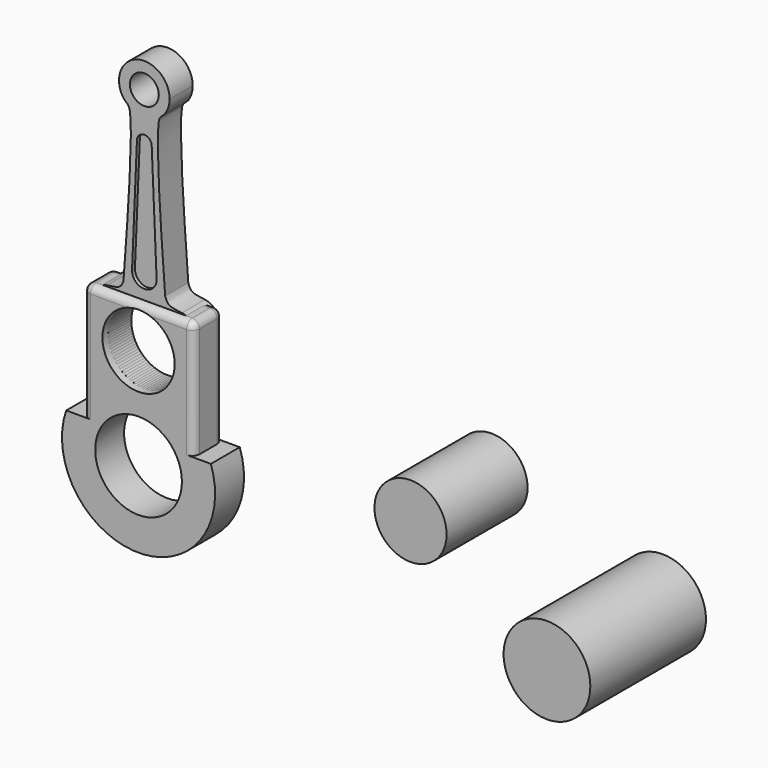
from build123d import *

# Parameters (mm, degrees)
F0_R          = 10
F1_DEPTH      = 20
F3_DEPTH      = 20
F5_DEPTH      = 2.5
F7_DEPTH      = 2.5
F8_R          = 30
F8_R_2        = 25
F9_DEPTH      = 25
F10_R         = 24.95
F11_DEPTH     = 35
F12_R         = 30
F13_DEPTH     = 100
F14_T1_DEPTH  = 66.4988437295
F14_T3_DEPTH  = 76.3163360927
F14_T6_ANGLE  = 90
F14_T8_ANGLE  = 90
F14_T10_ANGLE = 90
F14_T12_ANGLE = 90
F15_T1_DEPTH  = 69.8025602819


# Not quite as in the source:
# - a fillet or chamfer that OpenCascade refuses, or shapes differently, is made with other operations: its cross-section is extruded or revolved along the edge and cut away or added


with BuildPart() as f1:
    # F0 (on Front) → F1 (new body)
    with BuildSketch(Plane.XZ):
        with BuildLine():
            ThreePointArc((10.657655781, -13.8803592624), (0, -17.5), (-10.657655781, -13.8803592624))
            add(Edge.make_bspline(
                [(-10.657655781, -13.8803592624), (-10.5697063214, -14.0734920796), (-7.4212070748, -22.3661273448), (-11.0149524319, -76.0143110226), (-14.4087837187, -120.986558497)],
                knots=[0.171455294, 0.171455294, 0.171455294, 0.171455294, 0.1930861601, 1, 1, 1, 1], degree=3))
            add(Edge.make_bspline(
                [(-14.4087837187, -120.986558497), (-15, -122.5373980972), (-16.0166076681, -126.7545271526), (-23.3016373721, -127.0844308904), (-25.8878060456, -127.5592148304)],
                knots=[0, 0, 0, 0, 0.4297687598, 1, 1, 1, 1], degree=3))
            Line((-25.8878060456, -127.5592148304), (-35, -127.5592148304))
            Line((-35, -127.5592148304), (-35, -157.0267379284))
            Line((-35, -157.0267379284), (-25, -157.0267379284))
            ThreePointArc((-25, -157.0267379284), (0, -132.0267379284), (25, -157.0267379284))
            Line((25, -157.0267379284), (35, -157.0267379284))
            Line((35, -157.0267379284), (35, -127.5592148304))
            Line((35, -127.5592148304), (25.8878060456, -127.5592148304))
            add(Edge.make_bspline(
                [(14.4087837187, -120.986558497), (15, -122.5373980972), (16.0166076681, -126.7545271526), (23.3016373721, -127.0844308904), (25.8878060456, -127.5592148304)],
                knots=[0, 0, 0, 0, 0.4297687598, 1, 1, 1, 1], degree=3))
            add(Edge.make_bspline(
                [(10.657655781, -13.8803592624), (10.5697063214, -14.0734920796), (7.4212070748, -22.3661273448), (11.0149524319, -76.0143110226), (14.4087837187, -120.986558497)],
                knots=[0.171455294, 0.171455294, 0.171455294, 0.171455294, 0.1930861601, 1, 1, 1, 1], degree=3))
        make_face()
        with BuildLine():
            ThreePointArc((14.4087837187, -9.9316137535), (16.7093344433, -5.2007828701), (17.5, 0))
            ThreePointArc((17.5, 0), (-5.2007828701, 16.7093344433), (-14.4087837187, -9.9316137535))
            add(Edge.make_bspline(
                [(-14.4087837187, -9.9316137535), (-12.4132538877, -12.2865411794), (-11.3547799907, -12.3495077572), (-10.657655781, -13.8803592624)],
                knots=[0, 0, 0, 0, 0.171455294, 0.171455294, 0.171455294, 0.171455294], degree=3))
            ThreePointArc((-10.657655781, -13.8803592624), (0, -17.5), (10.657655781, -13.8803592624))
            add(Edge.make_bspline(
                [(14.4087837187, -9.9316137535), (12.4132538877, -12.2865411794), (11.3547799907, -12.3495077572), (10.657655781, -13.8803592624)],
                knots=[0, 0, 0, 0, 0.171455294, 0.171455294, 0.171455294, 0.171455294], degree=3))
        make_face()
        Circle(F0_R, mode=Mode.SUBTRACT)
    extrude(amount=F1_DEPTH)

    # F4 (on face) → F5 (cut)
    with BuildSketch(Plane.XZ.offset(20)):
        with BuildLine():
            Line((8.518111892, -113.2010370493), (5.076522479, -31.7173634542))
            ThreePointArc((5.076522479, -31.7173634542), (0, -27.4765780007), (-5.076522479, -31.7173634542))
            Line((-5.076522479, -31.7173634542), (-8.518111892, -113.2010370493))
            ThreePointArc((-8.518111892, -113.2010370493), (0, -121.3833500151), (8.518111892, -113.2010370493))
        make_face()
    extrude(amount=-F5_DEPTH, mode=Mode.SUBTRACT)

    # F6 (on face) → F7 (cut)
    with BuildSketch(Plane.XZ):
        with BuildLine():
            Line((8.518111892, -113.2010370493), (5.076522479, -31.7173634542))
            ThreePointArc((5.076522479, -31.7173634542), (0, -27.4765780007), (-5.076522479, -31.7173634542))
            Line((-5.076522479, -31.7173634542), (-8.518111892, -113.2010370493))
            ThreePointArc((-8.518111892, -113.2010370493), (0, -121.3833500151), (8.518111892, -113.2010370493))
        make_face()
    extrude(amount=F7_DEPTH, mode=Mode.SUBTRACT)

    # F15: fillet of radius 10 on 2 edges, made by hand

    # F15_s2 → F15_t1 (cut)
    with BuildSketch(Plane.XZ.offset(-24.901280141)):
        with BuildLine():
            ThreePointArc((35, -137.5197268868), (32.3782809806, -130.769840238), (25.8878060456, -127.5592148304))
            Line((25.8878060456, -127.5592148304), (35, -127.5592148304))
            Line((35, -127.5592148304), (35, -137.5197268868))
        make_face()
        with BuildLine():
            ThreePointArc((-35, -137.5197268868), (-32.3782809806, -130.769840238), (-25.8878060456, -127.5592148304))
            Line((-25.8878060456, -127.5592148304), (-35, -127.5592148304))
            Line((-35, -127.5592148304), (-35, -137.5197268868))
        make_face()
    extrude(amount=F15_T1_DEPTH, mode=Mode.SUBTRACT)


with BuildPart() as f3:
    # F2 (on Front) → F3 (new body)
    with BuildSketch(Plane.XZ):
        with BuildLine():
            ThreePointArc((25, -157.0267379284), (0, -182.0267379284), (-25, -157.0267379284))
            Line((-25, -157.0267379284), (-35, -157.0267379284))
            ThreePointArc((-35, -157.0267379284), (-32.403703492, -170.2554944837), (-25, -181.5216353562))
            ThreePointArc((-25, -181.5216353562), (0, -192.0267379284), (25, -181.5216353562))
            ThreePointArc((25, -181.5216353562), (32.403703492, -170.2554944837), (35, -157.0267379284))
            Line((35, -157.0267379284), (25, -157.0267379284))
        make_face()
        with BuildLine():
            ThreePointArc((-25, -181.5216353562), (-32.403703492, -170.2554944837), (-35, -157.0267379284))
            Line((-35, -157.0267379284), (-35, -181.5216353562))
            Line((-35, -181.5216353562), (-25, -181.5216353562))
        make_face()
        with BuildLine():
            Line((35, -181.5216353562), (35, -157.0267379284))
            ThreePointArc((35, -157.0267379284), (32.403703492, -170.2554944837), (25, -181.5216353562))
            Line((25, -181.5216353562), (35, -181.5216353562))
        make_face()
    extrude(amount=F3_DEPTH)


with BuildPart() as f9:
    # F8 (on Front) → F9 (new body)
    with BuildSketch(Plane.XZ):
        with BuildLine():
            ThreePointArc((38.2494218647, -133.2929936077), (36.7849557707, -129.7574597018), (33.2494218647, -128.2929936077))
            Line((33.2494218647, -128.2929936077), (-33.2494218647, -128.2929936077))
            ThreePointArc((-33.2494218647, -128.2929936077), (-36.7849557707, -129.7574597018), (-38.2494218647, -133.2929936077))
            Line((-38.2494218647, -133.2929936077), (-38.2494218647, -209.6093297005))
            Line((-38.2494218647, -209.6093297005), (-50.0230118632, -209.6093297005))
            ThreePointArc((-50.0230118632, -209.6093297005), (0, -279.9952929894), (50.0230118632, -209.6093297005))
            Line((50.0230118632, -209.6093297005), (38.2494218647, -209.6093297005))
            Line((38.2494218647, -209.6093297005), (38.2494218647, -133.2929936077))
        make_face()
        with Locations((0, -227.0267379284)):
            Circle(F8_R, mode=Mode.SUBTRACT)
        with Locations((0, -157.0267379284)):
            Circle(F8_R_2, mode=Mode.SUBTRACT)
    extrude(amount=F9_DEPTH)

    # F14: fillet of radius 5 on 10 edges, made by hand

    # F14_s2 → F14_t1 (cut)
    with BuildSketch(Plane.YZ.offset(-33.2494218647)):
        with BuildLine():
            ThreePointArc((-5, -128.2929936077), (-1.4644660941, -129.7574597018), (0, -133.2929936077))
            Line((0, -133.2929936077), (0, -128.2929936077))
            Line((0, -128.2929936077), (-5, -128.2929936077))
        make_face()
        with BuildLine():
            ThreePointArc((-20, -128.2929936077), (-23.5355339059, -129.7574597018), (-25, -133.2929936077))
            Line((-25, -133.2929936077), (-25, -128.2929936077))
            Line((-25, -128.2929936077), (-20, -128.2929936077))
        make_face()
    extrude(amount=F14_T1_DEPTH, mode=Mode.SUBTRACT)

    # F14_s4 → F14_t3 (cut)
    with BuildSketch(Plane.XY.offset(-209.6093297005)):
        with BuildLine():
            ThreePointArc((38.2494218647, -5), (36.7849557707, -1.4644660941), (33.2494218647, 0))
            Line((33.2494218647, 0), (38.2494218647, 0))
            Line((38.2494218647, 0), (38.2494218647, -5))
        make_face()
        with BuildLine():
            ThreePointArc((38.2494218647, -20), (36.7849557707, -23.5355339059), (33.2494218647, -25))
            Line((33.2494218647, -25), (38.2494218647, -25))
            Line((38.2494218647, -25), (38.2494218647, -20))
        make_face()
        with BuildLine():
            ThreePointArc((-38.2494218647, -5), (-36.7849557707, -1.4644660941), (-33.2494218647, 0))
            Line((-33.2494218647, 0), (-38.2494218647, 0))
            Line((-38.2494218647, 0), (-38.2494218647, -5))
        make_face()
        with BuildLine():
            ThreePointArc((-38.2494218647, -20), (-36.7849557707, -23.5355339059), (-33.2494218647, -25))
            Line((-33.2494218647, -25), (-38.2494218647, -25))
            Line((-38.2494218647, -25), (-38.2494218647, -20))
        make_face()
    extrude(amount=F14_T3_DEPTH, mode=Mode.SUBTRACT)

    # F14_s5 → F14_t6 (revolve, cut)
    with BuildSketch(Plane.YZ.offset(-33.2494218647)):
        with BuildLine():
            ThreePointArc((-20, -128.2929936077), (-23.5355339059, -129.7574597018), (-25, -133.2929936077))
            Line((-25, -133.2929936077), (-25, -128.2929936077))
            Line((-25, -128.2929936077), (-20, -128.2929936077))
        make_face()
    revolve(axis=Axis((-33.2494218647, -25, -133.2929936077), (0, -1, 0)), revolution_arc=F14_T6_ANGLE, mode=Mode.SUBTRACT)

    # F14_s7 → F14_t8 (revolve, cut)
    with BuildSketch(Plane.XY.offset(-133.2929936077)):
        with BuildLine():
            ThreePointArc((38.2494218647, -5), (36.7849557707, -1.4644660941), (33.2494218647, 0))
            Line((33.2494218647, 0), (38.2494218647, 0))
            Line((38.2494218647, 0), (38.2494218647, -5))
        make_face()
    revolve(axis=Axis((33.2494218647, 0, -133.2929936077), (0, -1, 0)), revolution_arc=F14_T8_ANGLE, mode=Mode.SUBTRACT)

    # F14_s9 → F14_t10 (revolve, cut)
    with BuildSketch(Plane.XY.offset(-133.2929936077)):
        with BuildLine():
            ThreePointArc((38.2494218647, -20), (36.7849557707, -23.5355339059), (33.2494218647, -25))
            Line((33.2494218647, -25), (38.2494218647, -25))
            Line((38.2494218647, -25), (38.2494218647, -20))
        make_face()
    revolve(axis=Axis((33.2494218647, -25, -133.2929936077), (0, -1, 0)), revolution_arc=F14_T10_ANGLE, mode=Mode.SUBTRACT)

    # F14_s11 → F14_t12 (revolve, cut)
    with BuildSketch(Plane.YZ.offset(-33.2494218647)):
        with BuildLine():
            ThreePointArc((-5, -128.2929936077), (-1.4644660941, -129.7574597018), (0, -133.2929936077))
            Line((0, -133.2929936077), (0, -128.2929936077))
            Line((0, -128.2929936077), (-5, -128.2929936077))
        make_face()
    revolve(axis=Axis((-33.2494218647, 0, -133.2929936077), (0, -1, 0)), revolution_arc=F14_T12_ANGLE, mode=Mode.SUBTRACT)


with BuildPart() as f11:
    # F10 (on Front) → F11 (new body, symmetric)
    with BuildSketch(Plane.XZ):
        with Locations((196.160569787, -192.8511559963)):
            Circle(F10_R)
    extrude(amount=F11_DEPTH, both=True)


with BuildPart() as f13:
    # F12 (on Front) → F13 (new body)
    with BuildSketch(Plane.XZ):
        with Locations((342.5459861755, -209.6093297005)):
            Circle(F12_R)
    extrude(amount=F13_DEPTH)


solid = Compound([f1.part, f3.part, f9.part, f11.part, f13.part])
